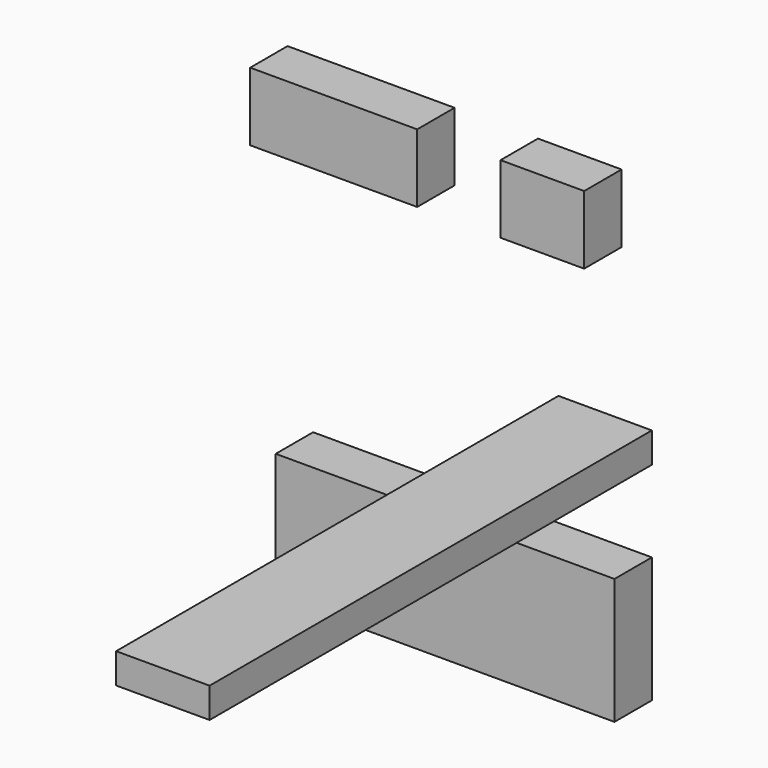
from build123d import *

# Parameters (mm, degrees)
F0_W     = 11.2635307014
F0_H     = 9.2887580395
F0_W_2   = 11.4305992611
F1_DEPTH = 6.35
F0_W_3   = 11.3646090031
F2_W     = 75.1274973154
F2_H     = 4.1087251157
F3_DEPTH = 12.7
F5_W     = 46.0354201496
F5_H     = 17.1042848378
F6_DEPTH = 6.35


# Not quite as in the source:
# - the program builds the solid bodies; features that only make, move or delete a surface that nothing else refers to are left out


with BuildPart() as f1:
    # F0 (on Front) → F1 (new body)
    with BuildSketch(Plane.XZ):
        with Locations((-43.8731033355, 57.5269795954)):
            Rectangle(F0_W, F0_H)
        with Locations((-32.5260383543, 57.5269795954)):
            Rectangle(F0_W_2, F0_H)
    extrude(amount=F1_DEPTH)


with BuildPart() as f1b:
    # F0 (on Front) → F1, piece 2 (new body)
    with BuildSketch(Plane.XZ):
        with Locations((-9.7989132628, 57.5269795954)):
            Rectangle(F0_W_3, F0_H)
    extrude(amount=F1_DEPTH)


with BuildPart() as f3:
    # F2 (on Right) → F3 (new body)
    with BuildSketch(Plane.YZ):
        with Locations((-37.5637486577, 30.2382716909)):
            Rectangle(F2_W, F2_H)
    extrude(amount=-F3_DEPTH)


with BuildPart() as f6:
    # F5 (on Front) → F6 (new body)
    with BuildSketch(Plane.XZ):
        with Locations((-23.0177100748, 8.5521424189)):
            Rectangle(F5_W, F5_H)
    extrude(amount=F6_DEPTH)


solid = Compound([f1.part, f1b.part, f3.part, f6.part])
